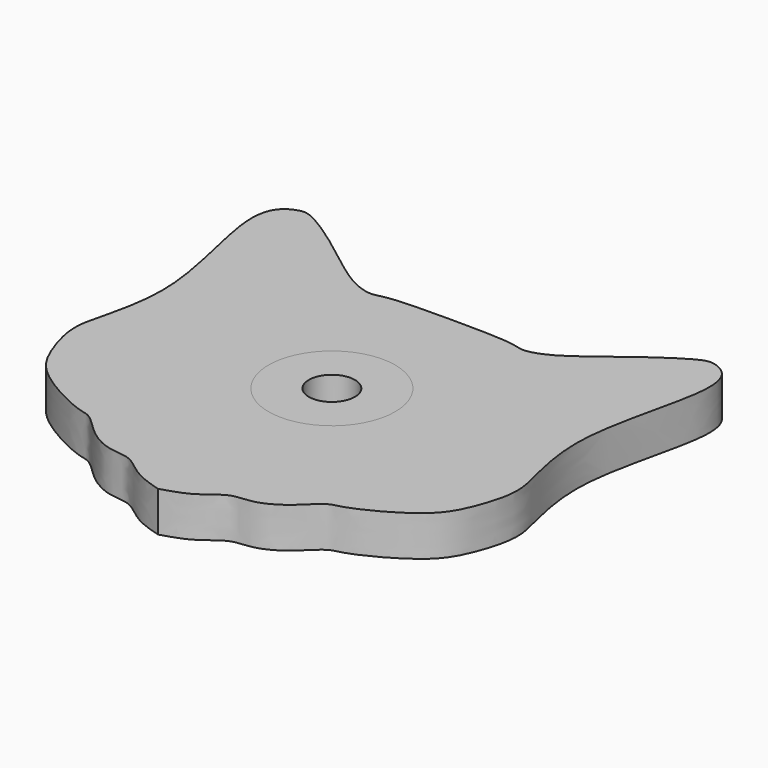
from build123d import *

# Parameters (mm, degrees)
F1_R     = 11
F1_R_2   = 4
F2_DEPTH = 7
F3_R     = 11
F4_DEPTH = 7


with BuildPart() as f2:
    # F1 (on Top) → F2 (new body)
    with BuildSketch(Plane.XY):
        Circle(F1_R)
        Circle(F1_R_2, mode=Mode.SUBTRACT)
    extrude(amount=F2_DEPTH)


with BuildPart() as f4:
    # F3 (on Top) → F4 (new body, through all)
    with BuildSketch(Plane.XY):
        with BuildLine():
            add(Edge.make_bspline(
                [(0, 25.8897617459), (4.3864055569, 25.8703153674), (10.8289101146, 25.8417536259), (13.2757002483, 24.6611704296), (17.8474108812, 26.2761901904), (23.594998976, 30.9202992901), (33.4937013261, 38.2138715063), (36.1675639167, 38.1806773323), (39.2855825143, 36.5848315949), (40.6715724711, 29.8977509674), (34.1473376422, 10.0883092219), (37.7336996012, -3.1394968098), (38.8698157184, -8.5086259705), (36.7537244866, -15.4845539707), (33.6701790157, -21.1369466388), (23.38847337, -26.5124231681), (20.5890565286, -26.5249775413), (17.1438835411, -30.5638448818), (12.6355944839, -33.0001390733), (8.5934381149, -32.6776161387), (5.0552641204, -36.2719007466), (1.7202712663, -37.2668030025), (0, -37.7799980342)],
                knots=[0, 0, 0, 0, 0.0656985275, 0.0964942838, 0.1366122657, 0.1933968461, 0.2619923062, 0.2926015893, 0.3258580246, 0.3741201394, 0.4650594165, 0.5378796558, 0.5831748819, 0.6344944194, 0.6862865162, 0.751805302, 0.784561497, 0.8284150022, 0.8732582997, 0.9115246968, 0.9543622644, 1, 1, 1, 1], degree=3))
            add(Edge.make_bspline(
                [(0, 25.8897617459), (-4.3864055569, 25.8703153674), (-10.8289101146, 25.8417536259), (-13.2757002483, 24.6611704296), (-17.8474108812, 26.2761901904), (-23.594998976, 30.9202992901), (-33.4937013261, 38.2138715063), (-36.1675639167, 38.1806773323), (-39.2855825143, 36.5848315949), (-40.6715724711, 29.8977509674), (-34.1473376422, 10.0883092219), (-37.7336996012, -3.1394968098), (-38.8698157184, -8.5086259705), (-36.7537244866, -15.4845539707), (-33.6701790157, -21.1369466388), (-23.38847337, -26.5124231681), (-20.5890565286, -26.5249775413), (-17.1438835411, -30.5638448818), (-12.6355944839, -33.0001390733), (-8.5934381149, -32.6776161387), (-5.0552641204, -36.2719007466), (-1.7202712663, -37.2668030025), (0, -37.7799980342)],
                knots=[0, 0, 0, 0, 0.0656985275, 0.0964942838, 0.1366122657, 0.1933968461, 0.2619923062, 0.2926015893, 0.3258580246, 0.3741201394, 0.4650594165, 0.5378796558, 0.5831748819, 0.6344944194, 0.6862865162, 0.751805302, 0.784561497, 0.8284150022, 0.8732582997, 0.9115246968, 0.9543622644, 1, 1, 1, 1], degree=3))
        make_face()
        Circle(F3_R, mode=Mode.SUBTRACT)
    extrude(amount=F4_DEPTH)


solid = Compound([f2.part, f4.part])
